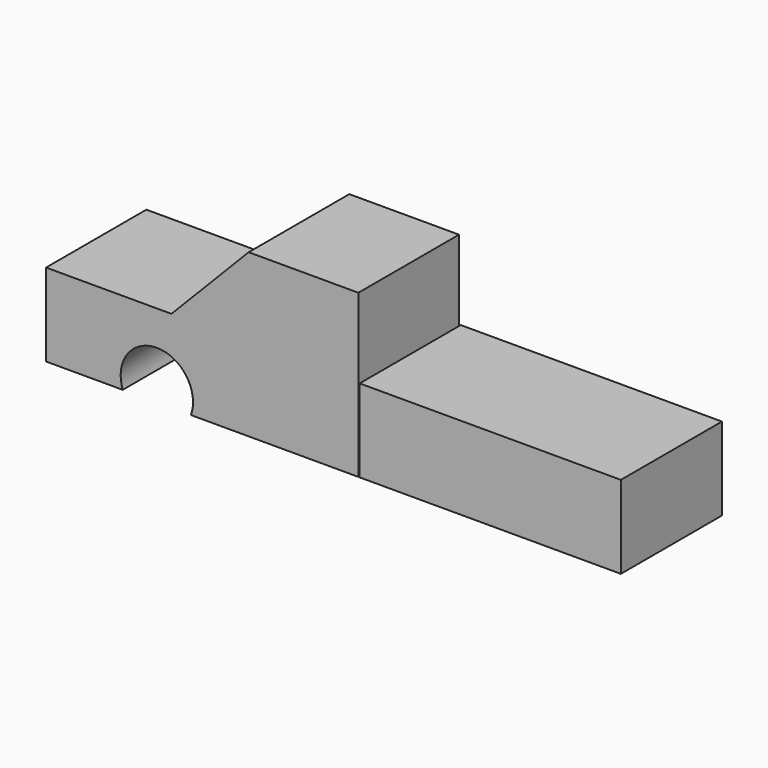
from build123d import *

# Parameters (mm, degrees)
F0_W          = 38.4747609496
F0_H          = 38.4747553617
F1_DEPTH      = 25.4
F3_DEPTH      = 38.608
F4_W          = 80.1557321101
F4_H          = 38.7662295252
F5_DEPTH      = 25.4
F7_DEPTH      = 210
F7_DEPTH_BACK = 127


# Not quite as in the source:
# - an extrude ends at something that could not be found from the text; its depth is read off the source's solid


with BuildPart() as f1:
    # F0 (on Top) → F1 (new body)
    with BuildSketch(Plane.XY):
        with Locations((-73.1603316963, -0.7286882028)):
            Rectangle(F0_W, F0_H)
    extrude(amount=-F1_DEPTH)

    # F2 (on face) → F3 (join)
    with BuildSketch(Plane.XZ.offset(19.9660658836)):
        Polygon((-53.9229512215, 0), (-53.9229512215, -25.4), (3.4455996938, -25.4), (3.4455996938, 24.3583643333), (-30.2235017333, 24.3583643333), align=None)
    extrude(amount=-F3_DEPTH)

    # F6 (on face) → F7 (cut, two sides)
    with BuildSketch(Plane.XZ.offset(19.9660658836)) as f7_sk:
        with BuildLine():
            ThreePointArc((-47.9401604074, -25.4), (-47.4690815305, -23.5841579821), (-47.3105455809, -21.7149164528))
            ThreePointArc((-47.3105455809, -21.7149164528), (-60.278839254, -10.7744002586), (-68.8790350419, -25.4))
            Line((-68.8790350419, -25.4), (-47.9401604074, -25.4))
        make_face()
    extrude(amount=F7_DEPTH, mode=Mode.SUBTRACT)
    extrude(f7_sk.sketch, amount=-F7_DEPTH_BACK, mode=Mode.SUBTRACT)


with BuildPart() as f5:
    # F4 (on Top) → F5 (new body)
    with BuildSketch(Plane.XY):
        with Locations((43.9295014367, -0.582951121)):
            Rectangle(F4_W, F4_H)
    extrude(amount=-F5_DEPTH)


solid = Compound([f1.part, f5.part])
